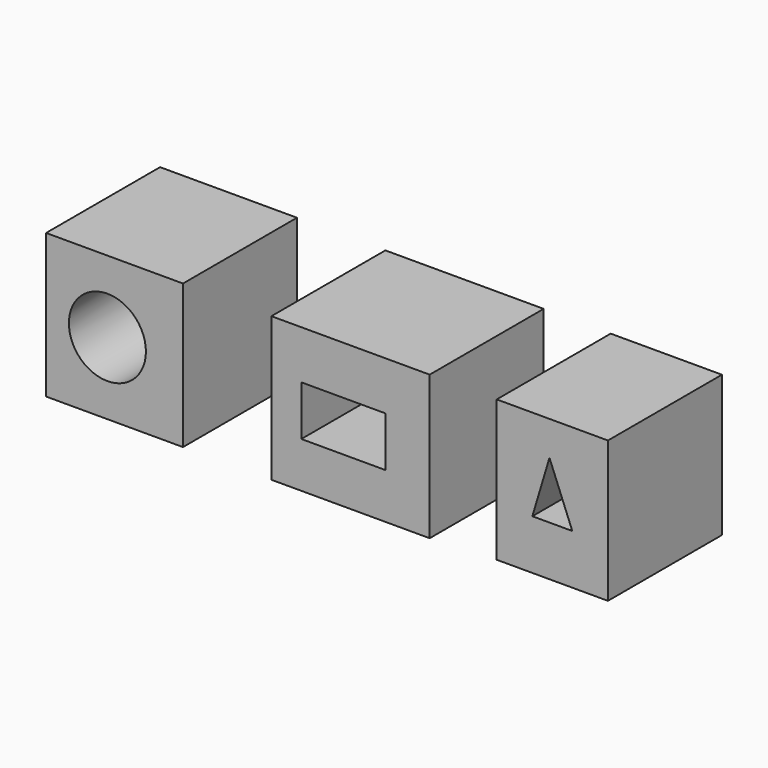
from build123d import *

# Parameters (mm, degrees)
F0_W      = 36.6095416248
F0_H      = 38.5162867606
F5_DEPTH  = 38.1
F2_W      = 42.3297788948
F2_H      = 38.5162867606
F6_DEPTH  = 38.1
F4_W      = 29.745247215
F4_H      = 37.7535894513
F7_DEPTH  = 38.1
F13_DEPTH = 12.7
F11_W     = 22.4996116012
F11_H     = 13.3472280577
F14_DEPTH = 50.8
F10_R     = 10.2964304388
F15_DEPTH = 25.4


# Not quite as in the source:
# - the program builds the solid bodies; features that only make, move or delete a surface that nothing else refers to are left out


with BuildPart() as f5:
    # F0 (on Front) → F5 (new body)
    with BuildSketch(Plane.XZ):
        with Locations((-57.9651016742, -19.2581433803)):
            Rectangle(F0_W, F0_H)
    extrude(amount=F5_DEPTH)

    # F10 (on face) → F15 (cut)
    with BuildSketch(Plane.XZ.offset(38.1)):
        with Locations((-59.8718486726, -19.2581433803)):
            Circle(F10_R)
    extrude(amount=-F15_DEPTH, mode=Mode.SUBTRACT)


with BuildPart() as f6:
    # F2 (on Front) → F6 (new body)
    with BuildSketch(Plane.XZ):
        with Locations((5.148219876, -19.2581433803)):
            Rectangle(F2_W, F2_H)
    extrude(amount=F6_DEPTH)

    # F11 (on face) → F14 (cut)
    with BuildSketch(Plane.XZ.offset(38.1)):
        with Locations((3.2414672896, -19.6394915693)):
            Rectangle(F11_W, F11_H)
    extrude(amount=-F14_DEPTH, mode=Mode.SUBTRACT)


with BuildPart() as f7:
    # F4 (on Front) → F7 (new body)
    with BuildSketch(Plane.XZ):
        with Locations((59.109153226, -18.8767947257)):
            Rectangle(F4_W, F4_H)
    extrude(amount=F7_DEPTH)

    # F12 (on face) → F13 (cut)
    with BuildSketch(Plane.XZ.offset(38.1)):
        Polygon((58.3464540541, -9.1523844749), (53.7702590227, -24.4063585997), (64.448043704, -24.4063585997), align=None)
    extrude(amount=-F13_DEPTH, mode=Mode.SUBTRACT)


solid = Compound([f5.part, f6.part, f7.part])
